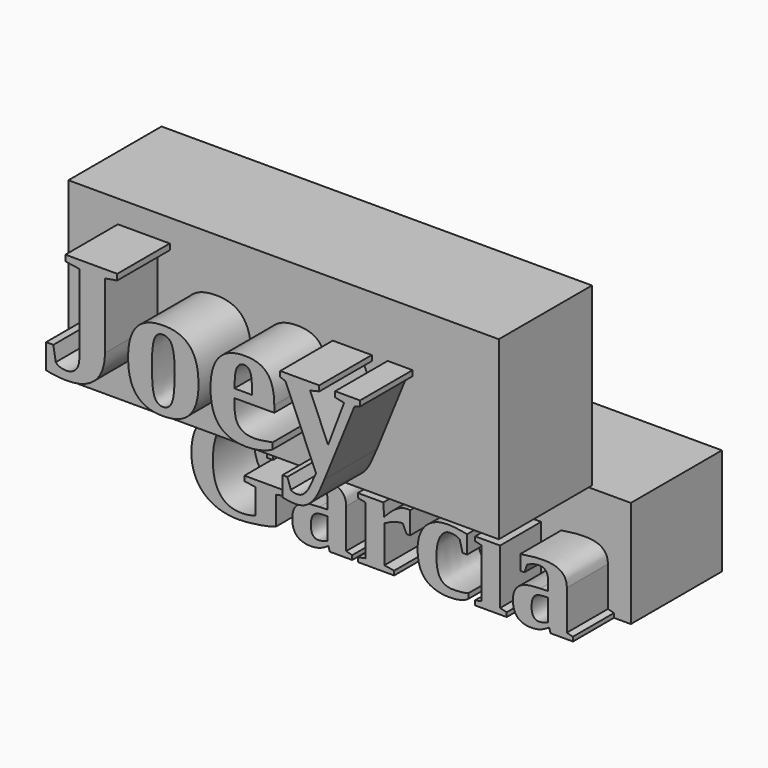
from build123d import *

# Parameters (mm, degrees)
F0_W         = 213.6698514223
F0_H         = 52.8256576508
F1_DEPTH     = 56.388
F2_TEXT_SIZE = 65.6152040594
F3_DEPTH     = 25.4
F4_W         = 213.1385356188
F4_H         = 65.1222020388
F5_DEPTH     = 57.658
F6_TEXT_SIZE = 82.2703871462
F7_DEPTH     = 32.512
F8_DEPTH     = 13.716
F9_DEPTH     = 8.382


# Not quite as in the source:
# - Text() gives the source's letters only with a copy of the font that has no kerning and outlines rounded to 1/6400 em; it was checked with that copy


with BuildPart() as f1:
    # F0 (on Front) → F1 (new body)
    with BuildSketch(Plane.XZ):
        with Locations((72.6546868682, -49.830772914)):
            Rectangle(F0_W, F0_H)
    extrude(amount=-F1_DEPTH)

    # F2 (on face) → F3 (join)
    with BuildSketch(Plane.XZ):
        with Locations((-21.0034754127, -76.2436017394)):
            Text('Garcia', F2_TEXT_SIZE, font='Tinos', font_style=FontStyle.BOLD, text_align=(TextAlign.LEFT, TextAlign.BOTTOM))
    extrude(amount=F3_DEPTH)


with BuildPart() as f5:
    # F4 (on Front) → F5 (new body)
    with BuildSketch(Plane.XZ):
        with Locations((53.6596253514, 32.5611010194)):
            Rectangle(F4_W, F4_H)
    extrude(amount=F5_DEPTH)

    # F6 (on face) → F7 (join)
    with BuildSketch(Plane.XZ.offset(57.658)):
        with Locations((-41.5972806513, 0)):
            Text('Joey', F6_TEXT_SIZE, font='Tinos', font_style=FontStyle.BOLD, text_align=(TextAlign.LEFT, TextAlign.BOTTOM))
    extrude(amount=F7_DEPTH)

    # F8 (add): a face of the model
    f8_faces = [f5.faces().sort_by_distance(p)[0] for p in [
        (53.6596253514, -28.829, 0),
    ]]
    extrude(f8_faces, amount=F8_DEPTH)

    # F9 (add): a face of the model
    f9_faces = [f5.faces().sort_by_distance(p)[0] for p in [
        (53.6596253514, -28.829, -13.716),
    ]]
    extrude(f9_faces, amount=F9_DEPTH)


solid = Compound([f1.part, f5.part])
